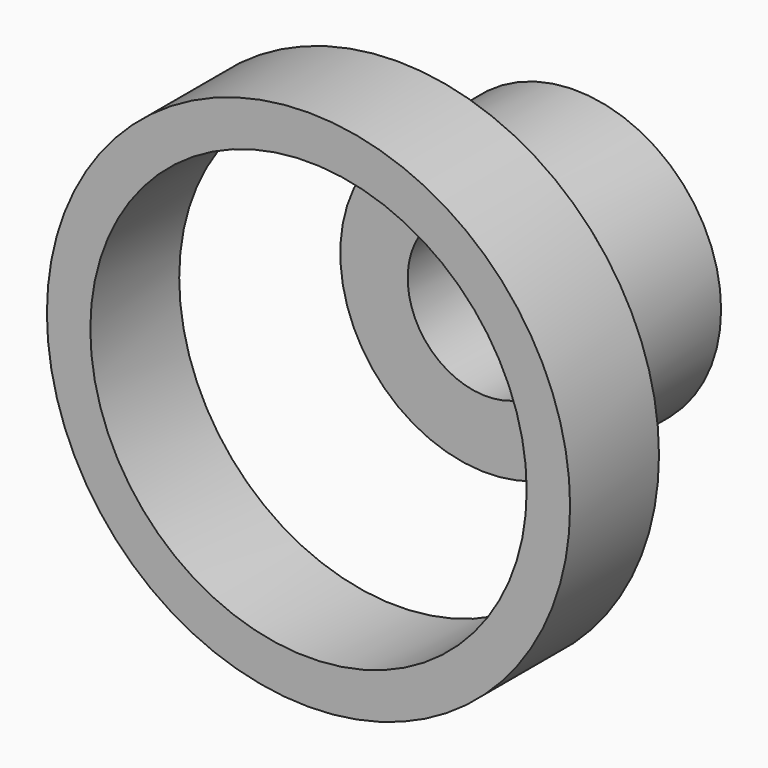
from build123d import *

# Parameters (mm, degrees)
F0_R     = 33.3720981505
F0_R_2   = 17.9593209069
F2_DEPTH = 25.4
F3_R     = 59.8115589421
F3_R_2   = 49.8848504809
F4_DEPTH = 25.4


# Not quite as in the source:
# - the program builds the solid bodies; features that only make, move or delete a surface that nothing else refers to are left out


with BuildPart() as f2:
    # F0 (on Front) → F2 (new body)
    with BuildSketch(Plane.XZ):
        Circle(F0_R)
        Circle(F0_R_2, mode=Mode.SUBTRACT)
    extrude(amount=F2_DEPTH)


with BuildPart() as f4:
    # F3 (on offset) → F4 (new body)
    with BuildSketch(Plane.XZ.offset(50.8)):
        Circle(F3_R)
        Circle(F3_R_2, mode=Mode.SUBTRACT)
    extrude(amount=F4_DEPTH)


solid = Compound([f2.part, f4.part])
